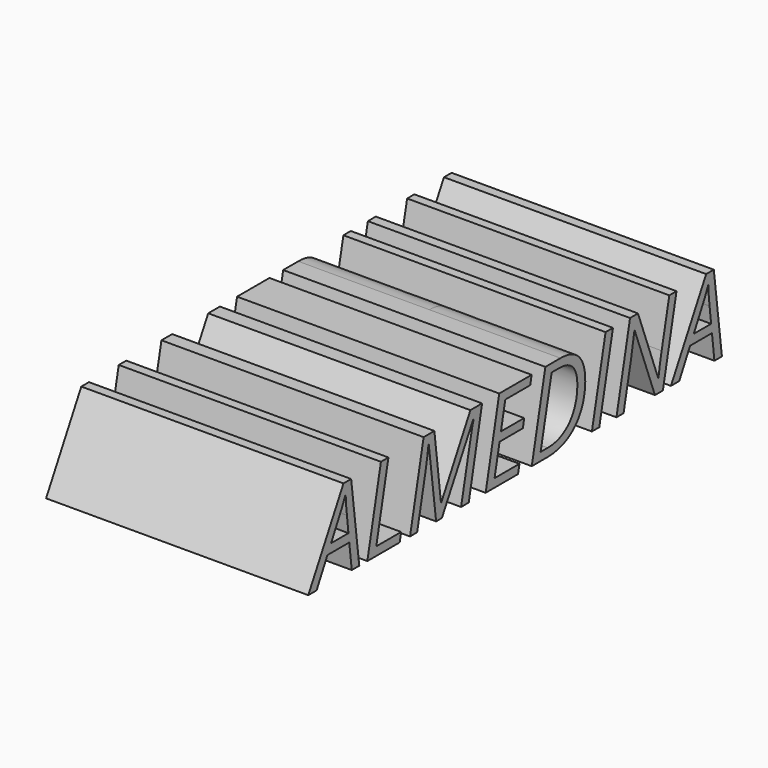
from build123d import *

# Parameters (mm, degrees)
F0_TEXT_SIZE = 21.512605042
F1_DEPTH     = 25


# Not quite as in the source:
# - Text() gives the source's letters only with a copy of the font that has no kerning and outlines rounded to 1/6400 em; it was checked with that copy


with BuildPart() as f1:
    # F0 (on Right) → F1 (new body, symmetric)
    with BuildSketch(Plane.YZ):
        with Locations((-35.6406756261, 13.1973231359)):
            Text('ALMEDINA', F0_TEXT_SIZE, font='Open Sans', font_style=FontStyle.ITALIC, text_align=(TextAlign.LEFT, TextAlign.BOTTOM))
    extrude(amount=F1_DEPTH, both=True)


solid = f1.part
